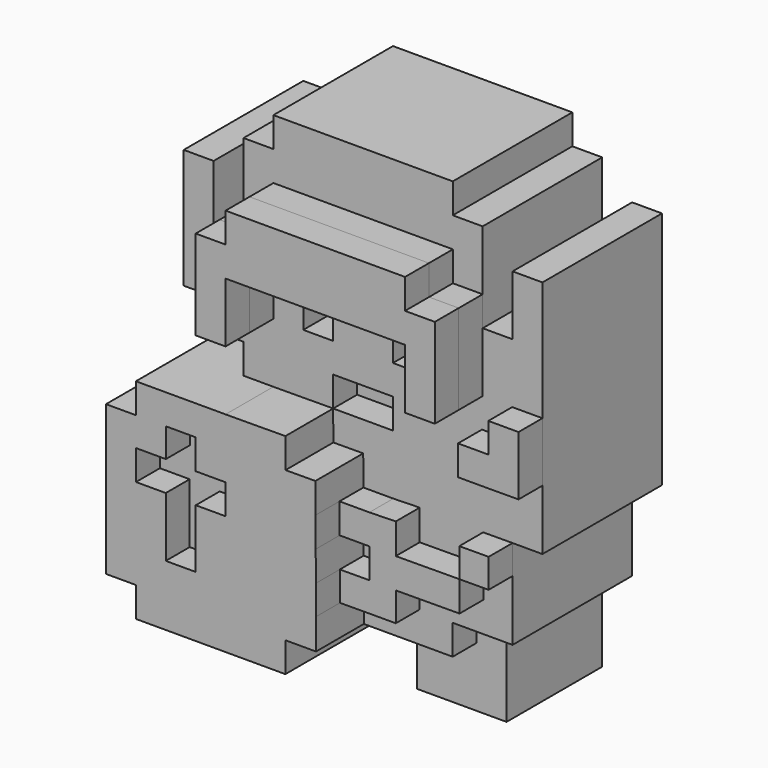
from build123d import *

# Parameters (mm, degrees)
F1_DEPTH = 12.7
F3_DEPTH = 5.08
F4_DEPTH = 2.54
F2_W     = 2.54
F2_H     = 5.08
F2_W_2   = 5.08
F2_H_2   = 2.54
F5_DEPTH = 2.54


# Not quite as in the source:
# - a feature names something its author has since deleted; it is built from what else it names


with BuildPart() as f1:
    # F0 (on Front) → F1 (new body)
    with BuildSketch(Plane.XZ):
        Polygon((2.285067299, 10.6943689859), (-12.954932701, 10.6943689859), (-12.954932701, 8.1543689859), (-15.494932701, 8.1543689859), (-15.494932701, 0.5343689859), (-18.034932701, 0.5343689859), (-18.034932701, 5.6143689859), (-20.574932701, 5.6143689859), (-20.574932701, -4.5456310141), (-18.034932701, -4.5456310141), (-18.034932701, -7.0856310141), (-15.494932701, -7.0856310141), (-15.494932701, -9.6256310141), (-20.574932701, -9.6256310141), (-20.574932701, -12.1656310141), (-23.114932701, -12.1656310141), (-23.114932701, -24.8656310141), (-20.574932701, -24.8656310141), (-20.574932701, -27.4056310141), (-7.874932701, -27.4056310141), (-7.874932701, -24.8656310141), (-2.794932701, -24.8656310141), (-2.794932701, -29.9456310141), (4.825067299, -29.9456310141), (4.825067299, -22.3256310141), (7.365067299, -22.3256310141), (7.365067299, -14.7056310141), (9.905067299, -14.7063690238), (9.905067299, 5.6136309762), (7.365067299, 5.6136309762), (7.365067299, 0.5343689859), (4.825067299, 0.5343689859), (4.825067299, 8.1543689859), (2.285067299, 8.1543689859), align=None)
    extrude(amount=F1_DEPTH)

    # F2 (on face) → F3 (join)
    with BuildSketch(Plane.XZ.offset(12.7)):
        Polygon((-12.954932701, -9.6256310141), (-15.494932701, -9.6256310141), (-20.574932701, -9.6256310141), (-20.574932701, -12.1656310141), (-23.114932701, -12.1656310141), (-23.114932701, -24.8656310141), (-20.574932701, -24.8656310141), (-20.574932701, -27.4056310141), (-7.874932701, -27.4056310141), (-7.874932701, -24.8656310141), (-5.2690269849, -24.8656310141), (-5.2690269849, -22.2557587346), (-5.2819938649, -19.7642921814), (-5.2952575954, -17.2157885193), (-5.3084768894, -14.6758229191), (-5.3217577861, -12.124020931), (-7.8617233863, -12.1372402251), (-7.874932701, -9.599192068), align=None)
        Polygon((-18.0264338851, -14.6206484801), (-18.0264338851, -12.1656310141), (-15.4883228242, -12.1656310141), (-15.4883228242, -14.7056310141), (-12.9483228242, -14.7056310141), (-12.9483228242, -17.2456310141), (-15.4883228242, -17.2456310141), (-15.4883228242, -22.2368724644), (-18.034932701, -22.2368724644), (-18.034932701, -17.1606484801), (-20.5664338851, -17.1606484801), (-20.5664338851, -14.6206484801), align=None, mode=Mode.SUBTRACT)
        Polygon((-12.954932701, 3.0743689859), (-15.494932701, 3.0743689859), (-15.494932701, 0.5343689859), (-15.494932701, -4.5456310141), (-12.954932701, -4.5456310141), (-12.954932701, 0.5343689859), (-10.414932701, 0.5343689859), (-7.874932701, 0.5343689859), (-2.7977656573, 0.5343689859), (-0.2577656573, 0.5343689859), (2.285067299, 0.5343689859), (2.285067299, -4.5456310141), (4.825067299, -4.5456310141), (4.825067299, 0.5343689859), (4.825067299, 3.0743689859), (2.2954009473, 3.0743689859), (2.2954009473, 5.6143689859), (-12.954932701, 5.6143689859), align=None)
    extrude(amount=F3_DEPTH)

    # F2 (on face) → F5 (cut)
    with BuildSketch(Plane.XZ.offset(12.7)):
        with Locations((-9.144932701, -2.0056310141)):
            Rectangle(F2_W, F2_H)
        with Locations((-1.5277656573, -2.0056310141)):
            Rectangle(F2_W, F2_H)
        with Locations((-5.334932701, -8.329192068)):
            Rectangle(F2_W_2, F2_H_2)
        Polygon((4.825067299, -24.8656310141), (4.825067299, -22.3256310141), (2.2784571629, -22.3256310141), (2.2784571629, -24.8656310141), (-2.794932701, -24.8656310141), (-2.794932701, -29.9456310141), (4.825067299, -29.9456310141), align=None)
    extrude(amount=-F5_DEPTH, mode=Mode.SUBTRACT)


with BuildPart() as f4:
    # F2 (on face) → F4 (new body)
    with BuildSketch(Plane.XZ.offset(12.7)):
        Polygon((-12.954932701, 3.0743689859), (-15.494932701, 3.0743689859), (-15.494932701, 0.5343689859), (-15.494932701, -4.5456310141), (-12.954932701, -4.5456310141), (-12.954932701, 0.5343689859), (-10.414932701, 0.5343689859), (-7.874932701, 0.5343689859), (-2.7977656573, 0.5343689859), (-0.2577656573, 0.5343689859), (2.285067299, 0.5343689859), (2.285067299, -4.5456310141), (4.825067299, -4.5456310141), (4.825067299, 0.5343689859), (4.825067299, 3.0743689859), (2.2954009473, 3.0743689859), (2.2954009473, 5.6143689859), (-12.954932701, 5.6143689859), align=None)
    extrude(amount=F4_DEPTH)


with BuildPart() as f4b:
    # F2 (on face) → F4, piece 2 (new body)
    with BuildSketch(Plane.XZ.offset(12.7)):
        Polygon((-15.4883228242, -12.1656310141), (-18.0264338851, -12.1656310141), (-18.0264338851, -14.6206484801), (-20.5664338851, -14.6206484801), (-20.5664338851, -17.1606484801), (-18.034932701, -17.1606484801), (-18.034932701, -22.2368724644), (-15.4883228242, -22.2368724644), (-15.4883228242, -17.2456310141), (-12.9483228242, -17.2456310141), (-12.9483228242, -14.7056310141), (-15.4883228242, -14.7056310141), align=None)
    extrude(amount=F4_DEPTH)


with BuildPart() as f4c:
    # F2 (on face) → F4, piece 3 (new body)
    with BuildSketch(Plane.XZ.offset(12.7)):
        Polygon((9.905067299, -9.585092935), (9.905067299, -4.5463690238), (7.3384868927, -4.5463690238), (7.3384868927, -7.0657309794), (4.7636916861, -7.0657309794), (4.7636916861, -9.5984507462), (7.3384868927, -9.5984507462), align=None)
    extrude(amount=F4_DEPTH)


with BuildPart() as f4d:
    # F2 (on face) → F4, piece 4 (new body)
    with BuildSketch(Plane.XZ.offset(12.7)):
        Polygon((7.365067299, -17.1747295235), (7.365067299, -14.7056310141), (4.8688458945, -14.7186226407), (4.8816287444, -17.1747295235), (4.8816960115, -17.1876542714), align=None)
    extrude(amount=F4_DEPTH)


with BuildPart() as f4e:
    # F2 (on face) → F4, piece 5 (new body)
    with BuildSketch(Plane.XZ.offset(12.7)):
        Polygon((-2.7684768894, -14.6758229191), (-5.3084768894, -14.6758229191), (-5.2952575954, -17.2157885193), (-2.7552575954, -17.2157885193), (-2.742062664, -19.7510730664), (-5.2819938649, -19.7642921814), (-5.2690269849, -22.2557587346), (-2.7288519475, -22.2425383505), (-0.5240406026, -22.2425383505), (-0.5240406026, -19.7799838678), (4.8950410482, -19.7517801655), (4.8816960115, -17.1876542714), (-0.5240406026, -17.2157885193), (-0.5240406026, -14.6225383505), align=None)
    extrude(amount=F4_DEPTH)


solid = Compound([f1.part, f4.part, f4b.part, f4c.part, f4d.part, f4e.part])
